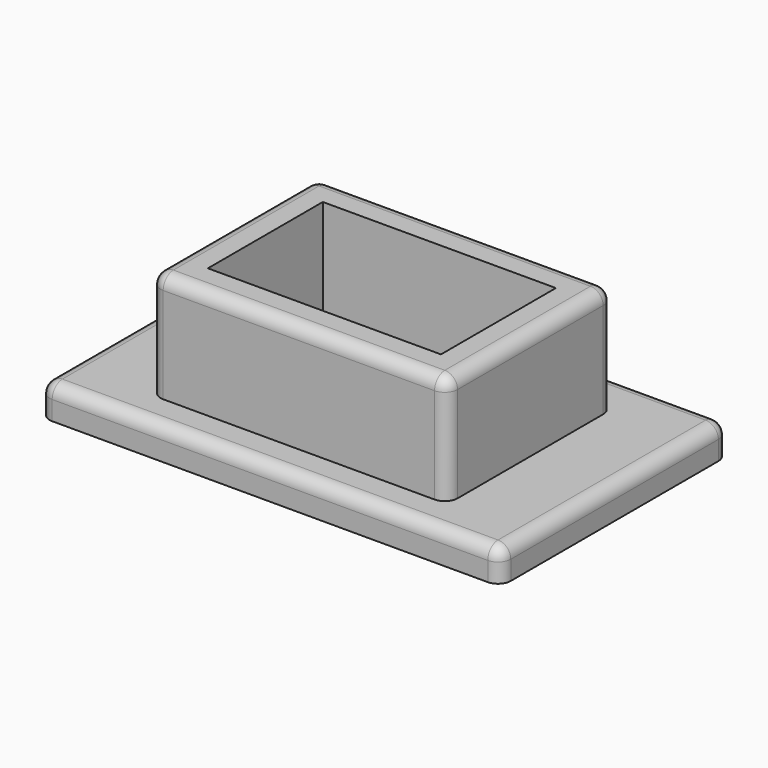
from build123d import *

# Parameters (mm, degrees)
F0_W     = 36.5
F0_H     = 22.5
F1_DEPTH = 17
F2_T     = 5
F3_W     = 8.5
F3_H     = 22.5
F4_DEPTH = 2
F0_W_2   = 72.2177475691
F0_H_2   = 44.6370989084
F5_DEPTH = 5
F6_R     = 2


# Not quite as in the source:
# - two fillets or chamfers of one size are made in one step


with BuildPart() as f1:
    # F0 (on Top) → F1 (new body)
    with BuildSketch(Plane.XY):
        with Locations((0.1048383191, -0.5443561636)):
            Rectangle(F0_W, F0_H)
    extrude(amount=F1_DEPTH)

    # F2
    f2_openings = [f1.faces().sort_by_distance(p)[0] for p in [
        (0.104838, -0.544356, 17),
    ]]
    offset(amount=F2_T, openings=f2_openings, kind=Kind.INTERSECTION)

    # F3 (on face) → F4 (cut)
    with BuildSketch(Plane.XY):
        with Locations((0.1048383191, -0.5443561636)):
            Rectangle(F3_W, F3_H)
    extrude(amount=-F4_DEPTH, mode=Mode.SUBTRACT)

    # F0 (on Top) → F5 (join)
    with BuildSketch(Plane.XY):
        Rectangle(F0_W_2, F0_H_2)
        with Locations((0.1048383191, -0.5443561636)):
            Rectangle(F0_W, F0_H, mode=Mode.SUBTRACT)
    extrude(amount=-F5_DEPTH)

    # F6
    f6_edges = [f1.edges().sort_by_distance(p)[0] for p in [
        (36.108874, -22.318549, -2.5),
        (36.108874, 22.318549, -2.5),
        (-36.108874, -22.318549, -2.5),
        (-36.108874, 22.318549, -2.5),
        (-23.145162, -0.544356, 17),
        (0.104838, -16.794356, 17),
        (23.354838, -0.544356, 17),
        (0.104838, 15.705644, 17),
        (-23.145162, -16.794356, 8.5),
        (-23.145162, 15.705644, 8.5),
        (23.354838, -16.794356, 8.5),
        (23.354838, 15.705644, 8.5),
        (0, 22.318549, 0),
        (36.108874, 0, 0),
        (-36.108874, 0, 0),
        (0, -22.318549, 0),
    ]]
    fillet(f6_edges, radius=F6_R)


solid = f1.part
